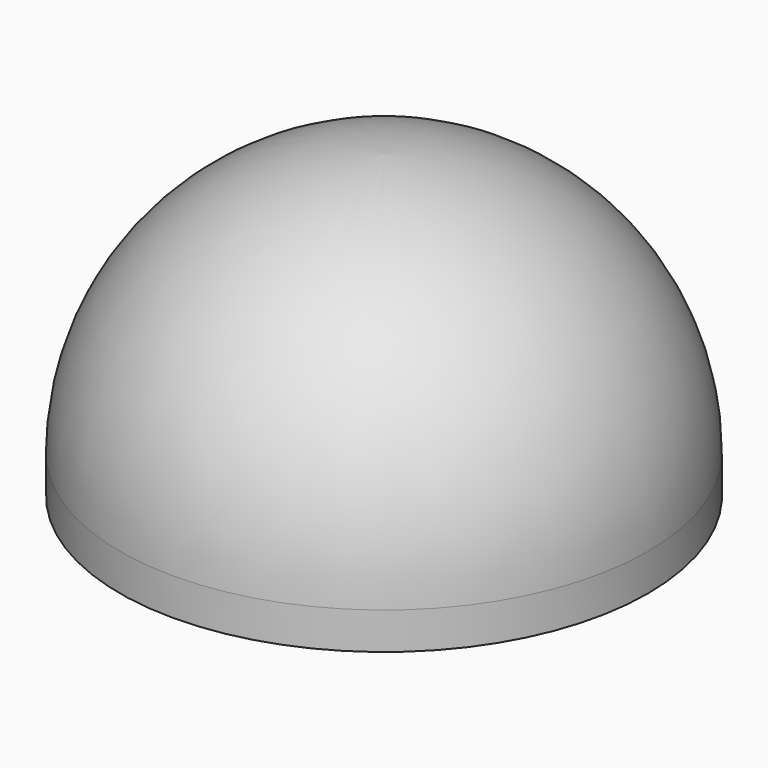
from build123d import *

# Parameters (mm, degrees)
F0_R          = 12.7
F1_DEPTH      = 11.938
F1_DEPTH_BACK = 2.54
F2_R          = 12.6999
F3_DEPTH      = 0.254


# Not quite as in the source:
# - a fillet or chamfer is up to 0.001 mm smaller than in the source, because OpenCascade refuses the exact size


with BuildPart() as f1:
    # F0 (on Top) → F1 (new body, two sides)
    with BuildSketch(Plane.XY) as f1_sk:
        with Locations((-47.3470948637, 36.0515639186)):
            Circle(F0_R)
    extrude(amount=F1_DEPTH)
    extrude(f1_sk.sketch, amount=-F1_DEPTH_BACK)

    # F2 (radius 12.7 in the source; OpenCascade refuses exactly that, so slightly less here)
    f2_edges = [f1.edges().sort_by_distance(p)[0] for p in [
        (-60.047095, 36.051564, 11.938),
    ]]
    fillet(f2_edges, radius=F2_R)

    # F3 (add): a face of the model
    f3_faces = [f1.faces().sort_by_distance(p)[0] for p in [
        (-47.3470948637, 36.0515639186, -2.54),
    ]]
    extrude(f3_faces, amount=-F3_DEPTH)


solid = f1.part
